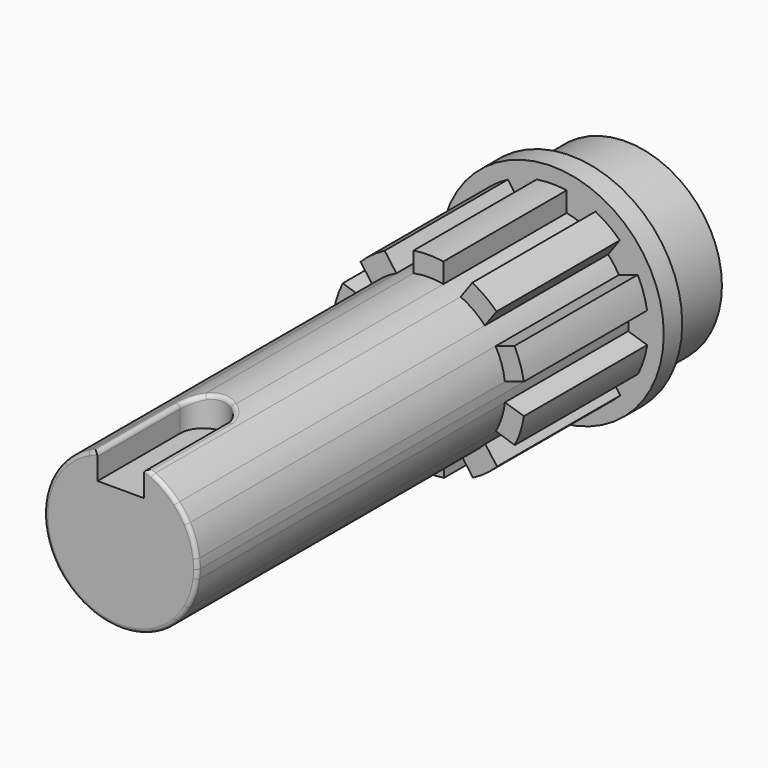
from build123d import *

# Parameters (mm, degrees)
F1_R     = 14.5
F1_R_2   = 12.45
F2_DEPTH = 3
F3_DEPTH = 12
F4_DEPTH = 20
F5_DEPTH = 70
F8_DEPTH = 25
F9_R     = 0.5


with BuildPart() as f2:
    # F1 (on Front) → F2 (new body)
    with BuildSketch(Plane.XZ):
        Circle(F1_R)
        Circle(F1_R_2, mode=Mode.SUBTRACT)
    extrude(amount=-F2_DEPTH)

    # F1 (on Front) → F3 (join)
    with BuildSketch(Plane.XZ):
        Circle(F1_R_2)
    extrude(amount=-F3_DEPTH)

    # F0 (on Front) → F4 (join)
    with BuildSketch(Plane.XZ):
        with BuildLine():
            ThreePointArc((-7.324554284, 6.7344936366), (-5.8782605878, 8.0279855793), (-4.2084272228, 9.0161876816))
            Line((-4.2084272228, 9.0161876816), (-5.7294038305, 11.1096323858))
            ThreePointArc((-5.7294038305, 11.1096323858), (-7.3861439392, 10.0843878203), (-8.8634461682, 8.8141546403))
            Line((-8.8634461682, 8.8141546403), (-7.324554284, 6.7344936366))
        make_face()
        with BuildLine():
            ThreePointArc((-1.9672528507, 9.7535847882), (-0.0368811837, 9.9499316469), (1.8948930083, 9.7679005158))
            Line((1.8948930083, 9.7679005158), (1.8948930083, 12.3555404773))
            ThreePointArc((1.8948930083, 12.3555404773), (-0.0480615306, 12.4999076032), (-1.9898484698, 12.3406038372))
            Line((-1.9898484698, 12.3406038372), (-1.9672528507, 9.7535847882))
        make_face()
        with BuildLine():
            ThreePointArc((4.141472307, 9.047138063), (5.818585579, 8.0713420111), (7.2744285153, 6.7886073517))
            Line((7.2744285153, 6.7886073517), (8.7954051229, 8.8820520559))
            ThreePointArc((8.7954051229, 8.8820520559), (7.3083787492, 10.140887538), (5.6438037116, 11.15336181))
            Line((5.6438037116, 11.15336181), (4.141472307, 9.047138063))
        make_face()
        with BuildLine():
            ThreePointArc((8.668295807, 4.8849920985), (9.4515504169, 3.1097740619), (9.8753795782, 1.2162969155))
            Line((9.8753795782, 1.2162969155), (12.3363714254, 2.015921639))
            ThreePointArc((12.3363714254, 2.015921639), (11.8732667494, 3.9083931094), (11.121714701, 5.7059146602))
            Line((11.121714701, 5.7059146602), (8.668295807, 4.8849920985))
        make_face()
        with BuildLine():
            Line((12.3515086878, -1.9209979529), (9.8841249332, -1.1430548127))
            ThreePointArc((9.8841249332, -1.1430548127), (9.474344242, -3.0396218816), (8.704271294, -4.820597602))
            Line((8.704271294, -4.820597602), (11.1652631412, -5.6202223254))
            ThreePointArc((11.1652631412, -5.6202223254), (11.9029704089, -3.8169746457), (12.3515086878, -1.9209979529))
        make_face()
        with BuildLine():
            Line((8.8634461682, -8.8141546403), (7.324554284, -6.7344936366))
            ThreePointArc((7.324554284, -6.7344936366), (5.8782605878, -8.0279855793), (4.2084272228, -9.0161876816))
            Line((4.2084272228, -9.0161876816), (5.7294038305, -11.1096323858))
            ThreePointArc((5.7294038305, -11.1096323858), (7.3861439392, -10.0843878203), (8.8634461682, -8.8141546403))
        make_face()
        with BuildLine():
            Line((1.9898484698, -12.3406038372), (1.9672528507, -9.7535847882))
            ThreePointArc((1.9672528507, -9.7535847882), (0.0368811837, -9.9499316469), (-1.8948930083, -9.7679005158))
            Line((-1.8948930083, -9.7679005158), (-1.8948930083, -12.3555404773))
            ThreePointArc((-1.8948930083, -12.3555404773), (0.0480615306, -12.4999076032), (1.9898484698, -12.3406038372))
        make_face()
        with BuildLine():
            Line((-5.6438037116, -11.15336181), (-4.141472307, -9.047138063))
            ThreePointArc((-4.141472307, -9.047138063), (-5.818585579, -8.0713420111), (-7.2744285153, -6.7886073517))
            Line((-7.2744285153, -6.7886073517), (-8.7954051229, -8.8820520559))
            ThreePointArc((-8.7954051229, -8.8820520559), (-7.3083787492, -10.140887538), (-5.6438037116, -11.15336181))
        make_face()
        with BuildLine():
            Line((-11.121714701, -5.7059146602), (-8.668295807, -4.8849920985))
            ThreePointArc((-8.668295807, -4.8849920985), (-9.4515504169, -3.1097740619), (-9.8753795782, -1.2162969155))
            Line((-9.8753795782, -1.2162969155), (-12.3363714254, -2.015921639))
            ThreePointArc((-12.3363714254, -2.015921639), (-11.8732667494, -3.9083931094), (-11.121714701, -5.7059146602))
        make_face()
        with BuildLine():
            ThreePointArc((-9.8841249332, 1.1430548127), (-9.474344242, 3.0396218816), (-8.704271294, 4.820597602))
            Line((-8.704271294, 4.820597602), (-11.1652631412, 5.6202223254))
            ThreePointArc((-11.1652631412, 5.6202223254), (-11.9029704089, 3.8169746457), (-12.3515086878, 1.9209979529))
            Line((-12.3515086878, 1.9209979529), (-9.8841249332, 1.1430548127))
        make_face()
    extrude(amount=F4_DEPTH)

    # F0 (on Front) → F5 (join)
    with BuildSketch(Plane.XZ):
        with BuildLine():
            ThreePointArc((9.8841249332, -1.1430548127), (9.9335175815, -0.5724757264), (9.95, 0))
            ThreePointArc((9.95, 0), (9.9313273736, 0.6092918829), (9.8753795782, 1.2162969155))
            ThreePointArc((9.8753795782, 1.2162969155), (9.4515504169, 3.1097740619), (8.668295807, 4.8849920985))
            ThreePointArc((8.668295807, 4.8849920985), (8.0279855793, 5.8782605878), (7.2744285153, 6.7886073517))
            ThreePointArc((7.2744285153, 6.7886073517), (5.818585579, 8.0713420111), (4.141472307, 9.047138063))
            ThreePointArc((4.141472307, 9.047138063), (3.0396218816, 9.474344242), (1.8948930083, 9.7679005158))
            ThreePointArc((1.8948930083, 9.7679005158), (-0.0368811837, 9.9499316469), (-1.9672528507, 9.7535847882))
            ThreePointArc((-1.9672528507, 9.7535847882), (-3.1097740619, 9.4515504169), (-4.2084272228, 9.0161876816))
            ThreePointArc((-4.2084272228, 9.0161876816), (-5.8782605878, 8.0279855793), (-7.324554284, 6.7344936366))
            ThreePointArc((-7.324554284, 6.7344936366), (-8.0713420111, 5.818585579), (-8.704271294, 4.820597602))
            ThreePointArc((-8.704271294, 4.820597602), (-9.474344242, 3.0396218816), (-9.8841249332, 1.1430548127))
            ThreePointArc((-9.8841249332, 1.1430548127), (-9.9499316469, -0.0368811837), (-9.8753795782, -1.2162969155))
            ThreePointArc((-9.8753795782, -1.2162969155), (-9.4515504169, -3.1097740619), (-8.668295807, -4.8849920985))
            ThreePointArc((-8.668295807, -4.8849920985), (-8.0279855793, -5.8782605878), (-7.2744285153, -6.7886073517))
            ThreePointArc((-7.2744285153, -6.7886073517), (-5.818585579, -8.0713420111), (-4.141472307, -9.047138063))
            ThreePointArc((-4.141472307, -9.047138063), (-3.0396218816, -9.474344242), (-1.8948930083, -9.7679005158))
            ThreePointArc((-1.8948930083, -9.7679005158), (0.0368811837, -9.9499316469), (1.9672528507, -9.7535847882))
            ThreePointArc((1.9672528507, -9.7535847882), (3.1097740619, -9.4515504169), (4.2084272228, -9.0161876816))
            ThreePointArc((4.2084272228, -9.0161876816), (5.8782605878, -8.0279855793), (7.324554284, -6.7344936366))
            ThreePointArc((7.324554284, -6.7344936366), (8.0713420111, -5.818585579), (8.704271294, -4.820597602))
            ThreePointArc((8.704271294, -4.820597602), (9.474344242, -3.0396218816), (9.8841249332, -1.1430548127))
        make_face()
    extrude(amount=F5_DEPTH)

    # F7 (on offset) → F8 (cut)
    with BuildSketch(Plane.XY.offset(6)):
        with BuildLine():
            Line((-3, -74.6025964618), (0, -74.6025964618))
            Line((0, -74.6025964618), (3, -74.6025964618))
            Line((3, -74.6025964618), (3, -56.6025964618))
            ThreePointArc((3, -56.6025964618), (0, -53.6025964618), (-3, -56.6025964618))
            Line((-3, -56.6025964618), (-3, -74.6025964618))
        make_face()
    extrude(amount=F8_DEPTH, mode=Mode.SUBTRACT)

    # F9
    f9_edges = [f2.edges().sort_by_distance(p)[0] for p in [
        (-3, -63.301298, 9.486965),
        (0, -53.602596, 9.95),
        (3, -63.301298, 9.486965),
        (-5.377611, -70, -8.371607),
        (7.65146, -70, 6.360634),
    ]]
    fillet(f9_edges, radius=F9_R)


solid = f2.part
